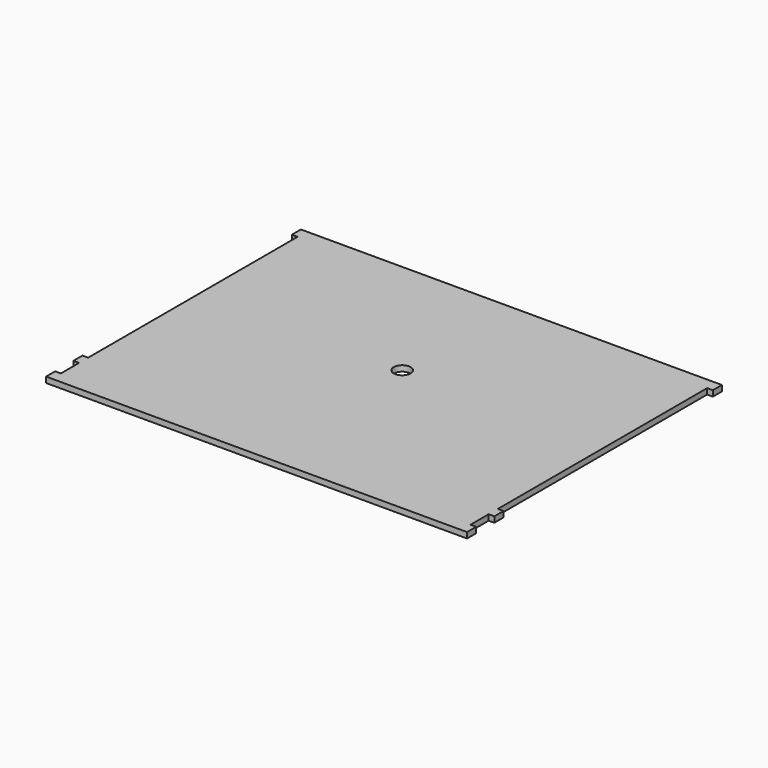
from build123d import *

# Parameters (mm, degrees)
F0_R     = 4.7625
F0_W     = 3.175
F0_H     = 6.35
F1_DEPTH = 3.175


# Not quite as in the source:
# - a length typed as a fraction of an inch, garbled in the dataset ("3 / 203.2 mm" for 3/8 in), is restored


with BuildPart() as f1:
    # F0 (on Top) → F1 (new body)
    with BuildSketch(Plane.XY):
        Polygon((228.6, 0), (0, 0), (0, -6.35), (0, -152.4), (0, -158.75), (0, -171.45), (0, -177.8), (228.6, -177.8), (228.6, -171.45), (228.6, -158.75), (228.6, -152.4), (228.6, -6.35), align=None)
        with Locations((114.3, -76.2)):
            Circle(F0_R, mode=Mode.SUBTRACT)
        with Locations((-1.5875, -155.575)):
            Rectangle(F0_W, F0_H)
        with Locations((-1.5875, -174.625)):
            Rectangle(F0_W, F0_H)
        with Locations((-1.5875, -3.175)):
            Rectangle(F0_W, F0_H)
        with Locations((230.1875, -3.175)):
            Rectangle(F0_W, F0_H)
        with Locations((230.1875, -155.575)):
            Rectangle(F0_W, F0_H)
        with Locations((230.1875, -174.625)):
            Rectangle(F0_W, F0_H)
    extrude(amount=F1_DEPTH)


solid = f1.part
